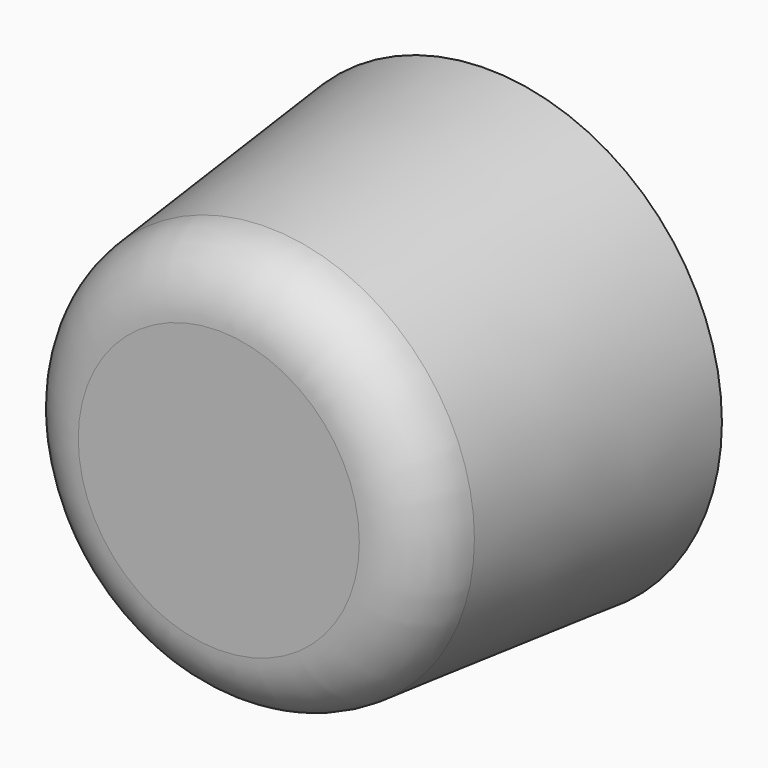
from build123d import *

# Parameters (mm, degrees)
F0_R     = 17.78
F2_R     = 15.24
F4_R     = 5.08
F5_R     = 11.1125
F6_DEPTH = 19.05


with BuildPart() as f3:
    # F0 (on Front) → F3 section 0
    with BuildSketch(Plane.XZ):
        Circle(F0_R)
    # F2 (on offset) → F3 section 1
    with BuildSketch(Plane.XZ.offset(25.4)):
        Circle(F2_R)
    loft()

    # F4
    f4_edges = [f3.edges().sort_by_distance(p)[0] for p in [
        (-15.24, -25.4, 0),
    ]]
    fillet(f4_edges, radius=F4_R)

    # F5 (on face) → F6 (cut)
    with BuildSketch(Plane(origin=(0, 0, 0), x_dir=(-1, 0, 0), z_dir=(0, 1, 0))):
        Circle(F5_R)
    extrude(amount=-F6_DEPTH, mode=Mode.SUBTRACT)


solid = f3.part
